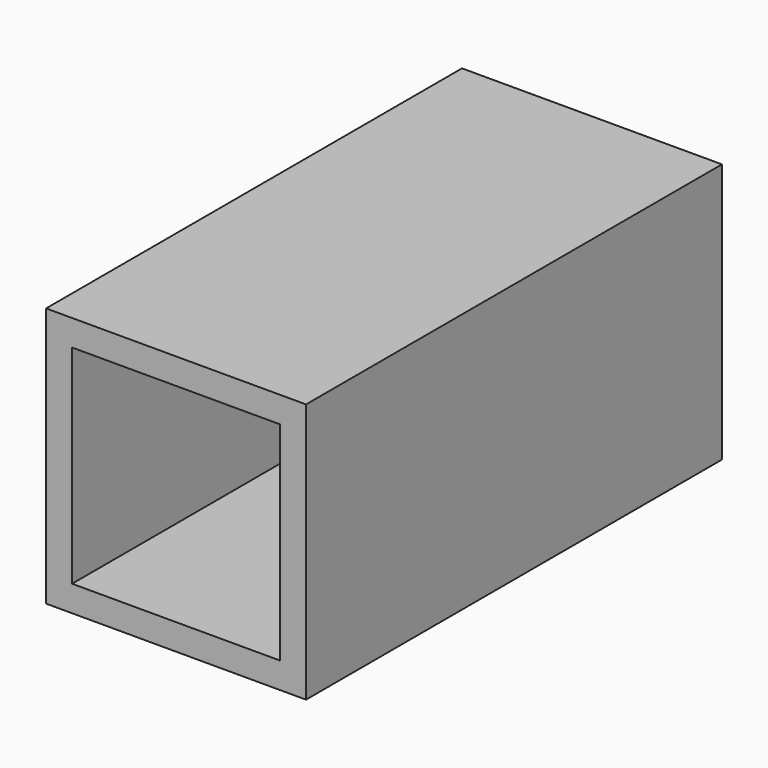
from build123d import *

# Parameters (mm, degrees)
F0_W     = 25.4
F0_H     = 25.4
F0_W_2   = 20.32
F0_H_2   = 20.32
F2_DEPTH = 50.8


# Not quite as in the source:
# - the program builds the solid bodies; features that only make, move or delete a surface that nothing else refers to are left out


with BuildPart() as f2:
    # F0 (on Front) → F2 (new body)
    with BuildSketch(Plane.XZ):
        Rectangle(F0_W, F0_H)
        Rectangle(F0_W_2, F0_H_2, mode=Mode.SUBTRACT)
    extrude(amount=F2_DEPTH)


solid = f2.part
